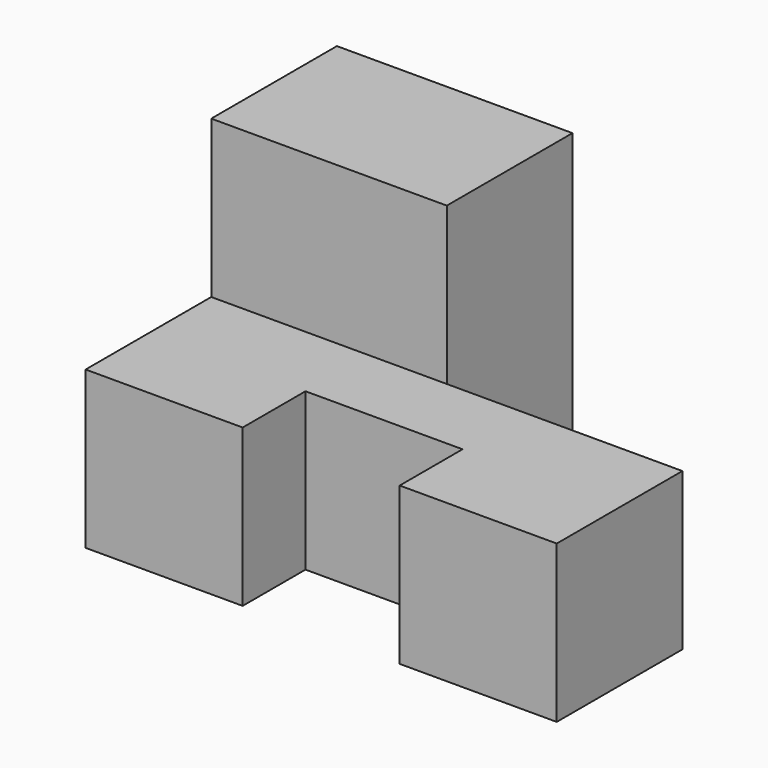
from build123d import *

# Parameters (mm, degrees)
F1_DEPTH = 20
F2_W     = 30
F2_H     = 20
F3_DEPTH = 40


with BuildPart() as f1:
    # F0 (on Top) → F1 (new body)
    with BuildSketch(Plane.XY):
        Polygon((-20, 0), (0, 0), (0, 20), (-60, 20), (-60, 0), (-40, 0), (-40, 10), (-20, 10), align=None)
    extrude(amount=F1_DEPTH)

    # F2 (on face) → F3 (join)
    with BuildSketch(Plane(origin=(0, 0, 0), x_dir=(1, 0, 0), z_dir=(0, 0, -1))):
        with Locations((-45, -30)):
            Rectangle(F2_W, F2_H)
    extrude(amount=-F3_DEPTH)


solid = f1.part
